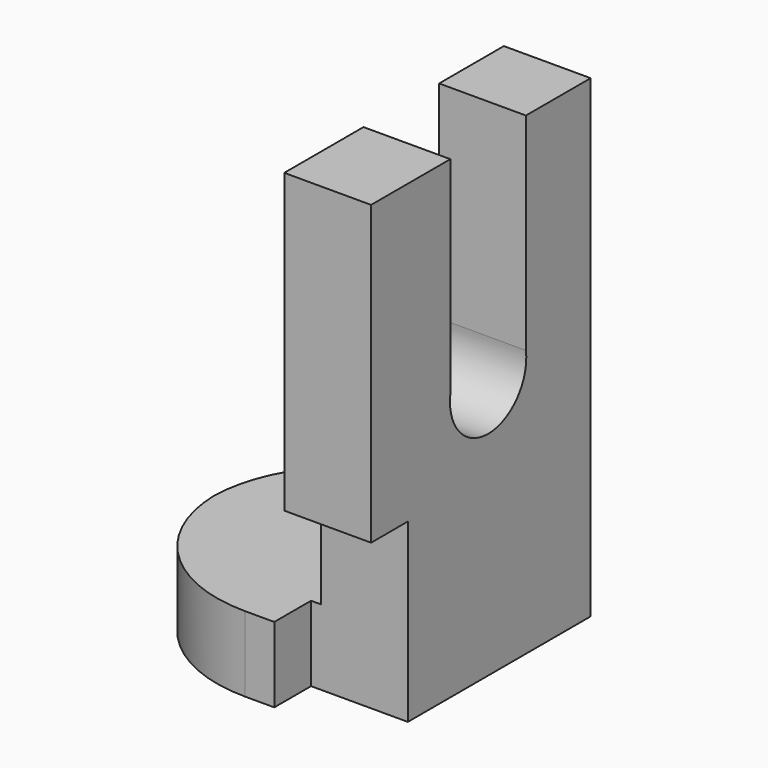
from build123d import *

# Parameters (mm, degrees)
F1_DEPTH    = 101.6
F2_T1_DEPTH = 288.460768654
F4_START    = 84.582
F3_W        = 46.8034986407
F3_H        = 78.1666617841
F4_DEPTH    = 39.37
F6_DEPTH    = 76.2


# Not quite as in the source:
# - a fillet or chamfer that OpenCascade refuses, or shapes differently, is made with other operations: its cross-section is extruded or revolved along the edge and cut away or added


with BuildPart() as f1:
    # F0 (on Front) → F1 (new body)
    with BuildSketch(Plane.XZ):
        Polygon((-46.8246676028, -52.1724224091), (51.9963987172, -52.1724224091), (51.9963987172, 123.2375688851), (19.8580101132, 123.2375688851), (19.8580101132, -24.3260078132), (-46.8246676028, -24.3260078132), align=None)
    extrude(amount=F1_DEPTH)

    # F2: fillet of radius 52.1228708116 on 2 edges, made by hand

    # F2_s2 → F2_t1 (cut)
    with BuildSketch(Plane.XY.offset(-182.4795994381)):
        with BuildLine():
            ThreePointArc((-46.8246676028, -52.1228708116), (-31.558232197, -15.2664354058), (5.2982032089, 0))
            Line((5.2982032089, 0), (-46.8246676028, 0))
            Line((-46.8246676028, 0), (-46.8246676028, -52.1228708116))
        make_face()
        with BuildLine():
            ThreePointArc((-46.8246676028, -49.4771291884), (-31.558232197, -86.3335645942), (5.2982032089, -101.6))
            Line((5.2982032089, -101.6), (-46.8246676028, -101.6))
            Line((-46.8246676028, -101.6), (-46.8246676028, -49.4771291884))
        make_face()
    extrude(amount=F2_T1_DEPTH, mode=Mode.SUBTRACT)

    # F3 (on Front) → F4 (cut)
    with BuildSketch(Plane.XZ.offset(F4_START)):
        with Locations((39.5658416674, -25.9385192767)):
            Rectangle(F3_W, F3_H)
    extrude(amount=F4_DEPTH, mode=Mode.SUBTRACT)

    # F5 (on Right) → F6 (cut, symmetric)
    with BuildSketch(Plane.YZ):
        with BuildLine():
            Line((-29.9497395754, 125.8109509945), (-64.9317279458, 125.8109509945))
            Line((-64.9317279458, 125.8109509945), (-64.9317279458, 46.6792732477))
            ThreePointArc((-64.9317279458, 46.6792732477), (-47.4407337606, 61.9233160809), (-29.9497395754, 46.6792732477))
            Line((-29.9497395754, 46.6792732477), (-29.9497395754, 125.8109509945))
        make_face()
        with BuildLine():
            ThreePointArc((-29.9497395754, 46.6792732477), (-47.4407337606, 61.9233160809), (-64.9317279458, 46.6792732477))
            ThreePointArc((-64.9317279458, 46.6792732477), (-48.6498471956, 26.6515784611), (-29.7841407761, 44.2667230964))
            ThreePointArc((-29.7841407761, 44.2667230964), (-29.8255891253, 45.4758365314), (-29.9497395754, 46.6792732477))
        make_face()
    extrude(amount=F6_DEPTH, both=True, mode=Mode.SUBTRACT)


solid = f1.part
